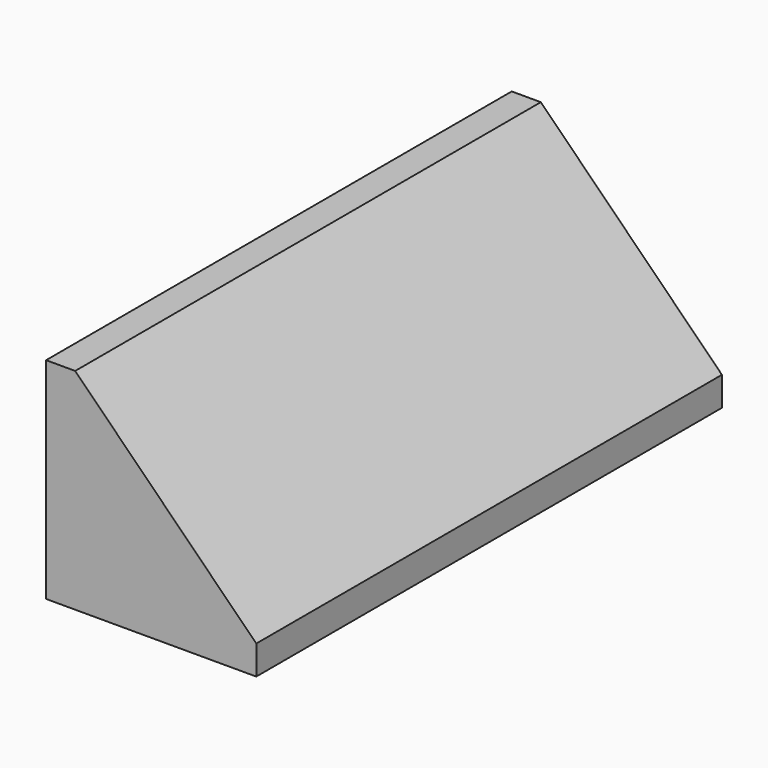
from build123d import *

# Parameters (mm, degrees)
F2_DEPTH = 127


# Not quite as in the source:
# - a variable given as a bare number and used for a length is read in inches; the dataset says mm whatever the document's units were


with BuildPart() as f2:
    # F1 (on Front) → F2 (new body)
    with BuildSketch(Plane.XZ):
        Polygon((-8.7344590575, 29.8639517277), (-15.0844590575, 29.8639517277), (-15.0844590575, -15.999175205), (30.7786678753, -15.999175205), (30.7786678753, -9.649175205), align=None)
    extrude(amount=F2_DEPTH)


solid = f2.part
